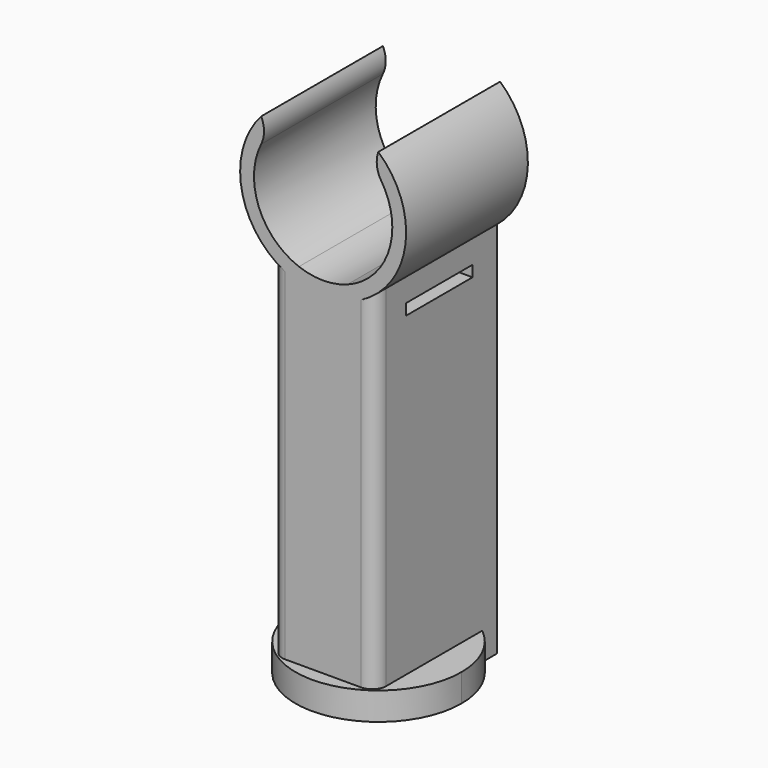
from build123d import *

# Parameters (mm, degrees)
F1_DEPTH    = 27.94
F3_DEPTH    = 50.8
F4_T1_DEPTH = 44.9110888614
F5_R        = 2.54
F6_W        = 15.24
F6_H        = 2.032
F7_DEPTH    = 25.4
F9_DEPTH    = 5.08
F10_DEPTH   = 5.08


# Not quite as in the source:
# - a fillet or chamfer that OpenCascade refuses, or shapes differently, is made with other operations: its cross-section is extruded or revolved along the edge and cut away or added


with BuildPart() as f1:
    # F0 (on Front) → F1 (new body)
    with BuildSketch(Plane.XZ):
        with BuildLine():
            ThreePointArc((-4.445, -11.8967211869), (-12.3269517561, -3.0555294801), (-9.4867838955, 8.4433957221))
            Line((-9.4867838955, 8.4433957221), (-11.3841406746, 10.1320748666))
            ThreePointArc((-11.3841406746, 10.1320748666), (-15.1860134607, -1.281637691), (-9.525, -11.8967211869))
            Line((-9.525, -11.8967211869), (-4.445, -11.8967211869))
        make_face()
        with BuildLine():
            Line((9.525, -11.8967211869), (4.445, -11.8967211869))
            ThreePointArc((4.445, -11.8967211869), (0, -12.7), (-4.445, -11.8967211869))
            Line((-4.445, -11.8967211869), (-9.525, -11.8967211869))
            ThreePointArc((-9.525, -11.8967211869), (0, -15.24), (9.525, -11.8967211869))
        make_face()
        with BuildLine():
            Line((9.525, -25.4), (9.525, -11.8967211869))
            ThreePointArc((9.525, -11.8967211869), (0, -15.24), (-9.525, -11.8967211869))
            Line((-9.525, -11.8967211869), (-9.525, -25.4))
            Line((-9.525, -25.4), (9.525, -25.4))
        make_face()
        with BuildLine():
            ThreePointArc((8.4433957221, 9.4867838955), (11.5870860373, 5.1989842435), (12.7, 0))
            ThreePointArc((12.7, 0), (10.4341147205, -7.2401139494), (4.445, -11.8967211869))
            Line((4.445, -11.8967211869), (9.525, -11.8967211869))
            ThreePointArc((9.525, -11.8967211869), (13.7371503595, -6.5991135768), (15.24, 0))
            ThreePointArc((15.24, 0), (13.9045032448, 6.2387810922), (10.1320748666, 11.3841406746))
            Line((10.1320748666, 11.3841406746), (8.4433957221, 9.4867838955))
        make_face()
    extrude(amount=F1_DEPTH)

    # F2 (on face) → F3 (join)
    with BuildSketch(Plane(origin=(0, 0, -25.4), x_dir=(1, 0, 0), z_dir=(0, 0, -1))):
        with BuildLine():
            Line((-9.525, 0), (-4.2597094971, 0))
            ThreePointArc((-4.2597094971, 0), (-7.0430625309, 1.175419304), (-9.525, 2.8983966834))
            Line((-9.525, 2.8983966834), (-9.525, 0))
        make_face()
        with BuildLine():
            Line((9.525, 2.8983966834), (9.525, 25.0416033166))
            ThreePointArc((9.525, 25.0416033166), (7.0430625309, 26.764580696), (4.2597094971, 27.94))
            Line((4.2597094971, 27.94), (-4.2597094971, 27.94))
            ThreePointArc((-4.2597094971, 27.94), (-7.0430625309, 26.764580696), (-9.525, 25.0416033166))
            Line((-9.525, 25.0416033166), (-9.525, 2.8983966834))
            ThreePointArc((-9.525, 2.8983966834), (-7.0430625309, 1.175419304), (-4.2597094971, 0))
            Line((-4.2597094971, 0), (4.2597094971, 0))
            ThreePointArc((4.2597094971, 0), (7.0430625309, 1.175419304), (9.525, 2.8983966834))
        make_face()
        with BuildLine():
            Line((9.525, 0), (9.525, 2.8983966834))
            ThreePointArc((9.525, 2.8983966834), (7.0430625309, 1.175419304), (4.2597094971, 0))
            Line((4.2597094971, 0), (9.525, 0))
        make_face()
        with BuildLine():
            ThreePointArc((-9.525, 25.0416033166), (-7.0430625309, 26.764580696), (-4.2597094971, 27.94))
            Line((-4.2597094971, 27.94), (-9.525, 27.94))
            Line((-9.525, 27.94), (-9.525, 25.0416033166))
        make_face()
        with BuildLine():
            ThreePointArc((4.2597094971, 27.94), (7.0430625309, 26.764580696), (9.525, 25.0416033166))
            Line((9.525, 25.0416033166), (9.525, 27.94))
            Line((9.525, 27.94), (4.2597094971, 27.94))
        make_face()
    extrude(amount=F3_DEPTH)

    # F4: fillet of radius 5.08 on 2 edges, made by hand

    # F4_s2 → F4_t1 (cut)
    with BuildSketch(Plane.XZ.offset(-8.4855444307)):
        with BuildLine():
            ThreePointArc((-11.3841406746, 10.1320748666), (-10.8580531921, 7.8805841193), (-11.3843237056, 5.6291361473))
            ThreePointArc((-11.3843237056, 5.6291361473), (-10.5299951264, 7.0999438475), (-9.4867838955, 8.4433957221))
            Line((-9.4867838955, 8.4433957221), (-11.3841406746, 10.1320748666))
        make_face()
        with BuildLine():
            ThreePointArc((10.1320748666, 11.3841406746), (9.8706902669, 9.0868255644), (10.6545556025, 6.9116166642))
            ThreePointArc((10.6545556025, 6.9116166642), (9.6353934931, 8.2734026998), (8.4433957221, 9.4867838955))
            Line((8.4433957221, 9.4867838955), (10.1320748666, 11.3841406746))
        make_face()
    extrude(amount=F4_T1_DEPTH, mode=Mode.SUBTRACT)

    # F5
    f5_edges = [f1.edges().sort_by_distance(p)[0] for p in [
        (-9.525, -27.94, -44.048361),
        (9.525, -27.94, -44.048361),
    ]]
    fillet(f5_edges, radius=F5_R)

    # F6 (on face) → F7 (cut)
    with BuildSketch(Plane.YZ.offset(9.525)):
        with Locations((-13.1727202785, -17.1660094585)):
            Rectangle(F6_W, F6_H)
    extrude(amount=-F7_DEPTH, mode=Mode.SUBTRACT)

    # F8 (on face) → F9 (join)
    with BuildSketch(Plane(origin=(0, 0, -76.2), x_dir=(1, 0, 0), z_dir=(0, 0, -1))):
        with BuildLine():
            ThreePointArc((9.525, 3.3432788131), (13.7371503595, 8.6408864232), (15.24, 15.24))
            ThreePointArc((15.24, 15.24), (-6.5991135768, 28.9771503595), (-9.525, 3.3432788131))
            Line((-9.525, 3.3432788131), (-9.525, 25.4))
            ThreePointArc((-9.525, 25.4), (-8.7810512242, 27.1960512242), (-6.985, 27.94))
            Line((-6.985, 27.94), (6.985, 27.94))
            ThreePointArc((6.985, 27.94), (8.7810512242, 27.1960512242), (9.525, 25.4))
            Line((9.525, 25.4), (9.525, 3.3432788131))
        make_face()
        with BuildLine():
            Line((-9.525, 25.4), (-9.525, 3.3432788131))
            ThreePointArc((-9.525, 3.3432788131), (-5.0473542134, 0.8600898666), (0, 0))
            ThreePointArc((0, 0), (5.0473542134, 0.8600898666), (9.525, 3.3432788131))
            Line((9.525, 3.3432788131), (9.525, 25.4))
            ThreePointArc((9.525, 25.4), (8.7810512242, 27.1960512242), (6.985, 27.94))
            Line((6.985, 27.94), (-6.985, 27.94))
            ThreePointArc((-6.985, 27.94), (-8.7810512242, 27.1960512242), (-9.525, 25.4))
        make_face()
    extrude(amount=F9_DEPTH)

    # F10 (add): faces of the model
    f10_faces = [f1.faces().sort_by_distance(p)[0] for p in [
        (-7.1991537336, -0.9808264472, -76.2),
        (7.1991537336, -0.9808264472, -76.2),
    ]]
    extrude(f10_faces, amount=F10_DEPTH)


solid = f1.part
